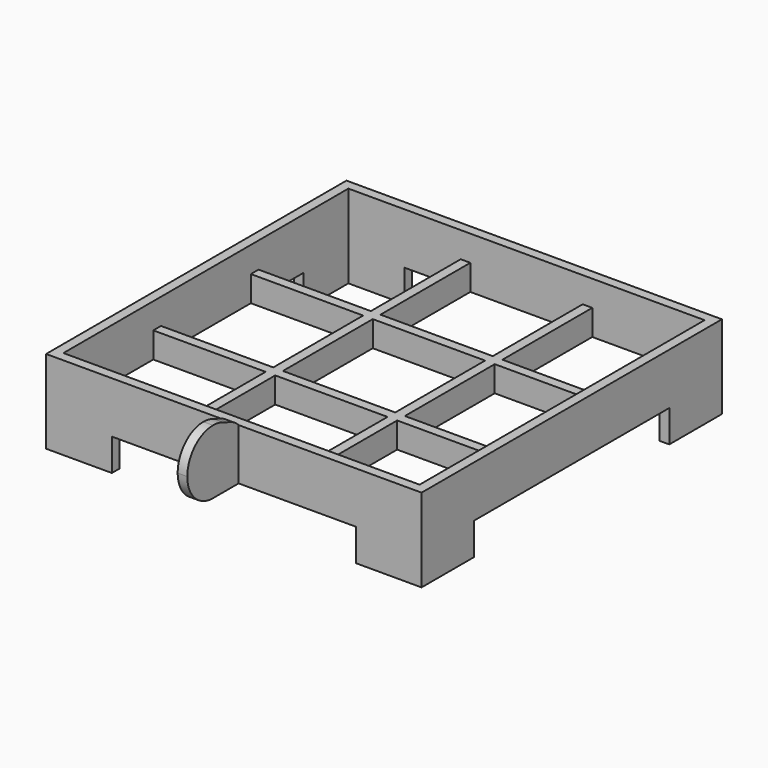
from build123d import *

# Parameters (mm, degrees)
F0_W        = 58.5
F0_H        = 58.5
F0_W_2      = 17.5
F0_H_2      = 17.5
F1_DEPTH    = 4
F2_W        = 1.5
F2_H        = 10
F3_DEPTH    = 10
F4_R        = 4.99999
F6_DEPTH    = 1.5
F7_T1_DEPTH = 26.0435355486
F8_R        = 5
F9_W        = 58.5
F9_H        = 58.5
F9_W_2      = 55.5
F9_H_2      = 55.5
F10_DEPTH   = 4
F12_DEPTH   = 5


# Not quite as in the source:
# - a fillet or chamfer that OpenCascade refuses, or shapes differently, is made with other operations: its cross-section is extruded or revolved along the edge and cut away or added
# - a fillet or chamfer is up to 0.001 mm smaller than in the source, because OpenCascade refuses the exact size


with BuildPart() as f1:
    # F0 (on Top) → F1 (new body)
    with BuildSketch(Plane.XY):
        with Locations((-13.779699502, 7.1240415001)):
            Rectangle(F0_W, F0_H)
        with Locations((-32.779699502, -11.8759584999)):
            Rectangle(F0_W_2, F0_H_2, mode=Mode.SUBTRACT)
        with Locations((-13.779699502, -11.8759584999)):
            Rectangle(F0_W_2, F0_H_2, mode=Mode.SUBTRACT)
        with Locations((5.220300498, -11.8759584999)):
            Rectangle(F0_W_2, F0_H_2, mode=Mode.SUBTRACT)
        with Locations((-32.779699502, 7.1240415001)):
            Rectangle(F0_W_2, F0_H_2, mode=Mode.SUBTRACT)
        with Locations((-32.779699502, 26.1240415001)):
            Rectangle(F0_W_2, F0_H_2, mode=Mode.SUBTRACT)
        with Locations((-13.779699502, 7.1240415001)):
            Rectangle(F0_W_2, F0_H_2, mode=Mode.SUBTRACT)
        with Locations((5.220300498, 7.1240415001)):
            Rectangle(F0_W_2, F0_H_2, mode=Mode.SUBTRACT)
        with Locations((-13.779699502, 26.1240415001)):
            Rectangle(F0_W_2, F0_H_2, mode=Mode.SUBTRACT)
        with Locations((5.220300498, 26.1240415001)):
            Rectangle(F0_W_2, F0_H_2, mode=Mode.SUBTRACT)
    extrude(amount=F1_DEPTH)

    # F2 (on face) → F3 (join)
    with BuildSketch(Plane.XZ.offset(22.1259584999)):
        with Locations((-13.779699502, 5)):
            Rectangle(F2_W, F2_H)
    extrude(amount=F3_DEPTH)

    # F4 (radius 5 in the source; OpenCascade refuses exactly that, so slightly less here)
    f4_edges = [f1.edges().sort_by_distance(p)[0] for p in [
        (-13.7797, -32.125958, 10),
        (-13.7797, -32.125958, 0),
        (-13.7797, -22.125958, 10),
    ]]
    fillet(f4_edges, radius=F4_R)

    # F5 (on face) → F6 (join)
    with BuildSketch(Plane(origin=(-14.529699502, 0, 0), x_dir=(0, -1, 0), z_dir=(-1, 0, 0))):
        with BuildLine():
            Line((20.6259584999, 4), (22.1259584999, 4))
            Line((22.1259584999, 4), (22.1259584999, 5))
            ThreePointArc((22.1259584999, 5), (22.8099724149, 7.5243343902), (24.6748641453, 9.3579968409))
            Line((24.6748641453, 9.3579968409), (22.1259584999, 9.3579968409))
            Line((22.1259584999, 9.3579968409), (20.6259584999, 9.3579968409))
            Line((20.6259584999, 9.3579968409), (20.6259584999, 4))
        make_face()
    extrude(amount=-F6_DEPTH)

    # F7: fillet of radius 5 on 1 edges, made by hand

    # F7_s2 → F7_t1 (cut)
    with BuildSketch(Plane.YZ.offset(-26.8014672763)):
        with BuildLine():
            ThreePointArc((-20.6259584999, 4.4492897311), (-21.7687892868, 7.6308374145), (-24.6748567646, 9.3579968409))
            Line((-24.6748567646, 9.3579968409), (-24.6558347299, 9.4561709831))
            ThreePointArc((-24.6558347299, 9.4561709831), (-22.6504076323, 9.4579968409), (-20.6259584999, 9.4579968409))
            Line((-20.6259584999, 9.4579968409), (-20.5259584999, 9.3579968409))
            Line((-20.5259584999, 9.3579968409), (-20.5259584999, 4.4492897311))
            Line((-20.5259584999, 4.4492897311), (-20.6259584999, 4.4492897311))
        make_face()
    extrude(amount=F7_T1_DEPTH, mode=Mode.SUBTRACT)

    # F8
    f8_edges = [f1.edges().sort_by_distance(p)[0] for p in [
        (-13.7797, -24.674857, 9.357997),
    ]]
    fillet(f8_edges, radius=F8_R)

    # F9 (on face) → F10 (join)
    with BuildSketch(Plane.XY.offset(4)):
        with Locations((-13.779699502, 7.1240415001)):
            Rectangle(F9_W, F9_H)
        with Locations((-13.779699502, 7.1240415001)):
            Rectangle(F9_W_2, F9_H_2, mode=Mode.SUBTRACT)
    extrude(amount=F10_DEPTH)

    # F11 (on face) → F12 (join)
    with BuildSketch(Plane(origin=(0, 0, 0), x_dir=(1, 0, 0), z_dir=(0, 0, -1))):
        Polygon((-43.029699502, 11.8759584999), (-41.529699502, 11.8759584999), (-41.529699502, 20.6259584999), (-32.779699502, 20.6259584999), (-32.779699502, 22.1259584999), (-41.529699502, 22.1259584999), (-43.029699502, 22.1259584999), align=None)
        Polygon((5.220300498, 22.1259584999), (5.220300498, 20.6259584999), (13.970300498, 20.6259584999), (13.970300498, 11.8759584999), (15.470300498, 11.8759584999), (15.470300498, 22.1259584999), (13.970300498, 22.1259584999), align=None)
        Polygon((-43.029699502, -36.3740415001), (-32.779699502, -36.3740415001), (-32.779699502, -34.8740415001), (-41.529699502, -34.8740415001), (-41.529699502, -26.1240415001), (-43.029699502, -26.1240415001), (-43.029699502, -34.8740415001), align=None)
        Polygon((13.970300498, -34.8740415001), (5.220300498, -34.8740415001), (5.220300498, -36.3740415001), (15.470300498, -36.3740415001), (15.470300498, -34.8740415001), (15.470300498, -26.1240415001), (13.970300498, -26.1240415001), align=None)
    extrude(amount=F12_DEPTH)


solid = f1.part
